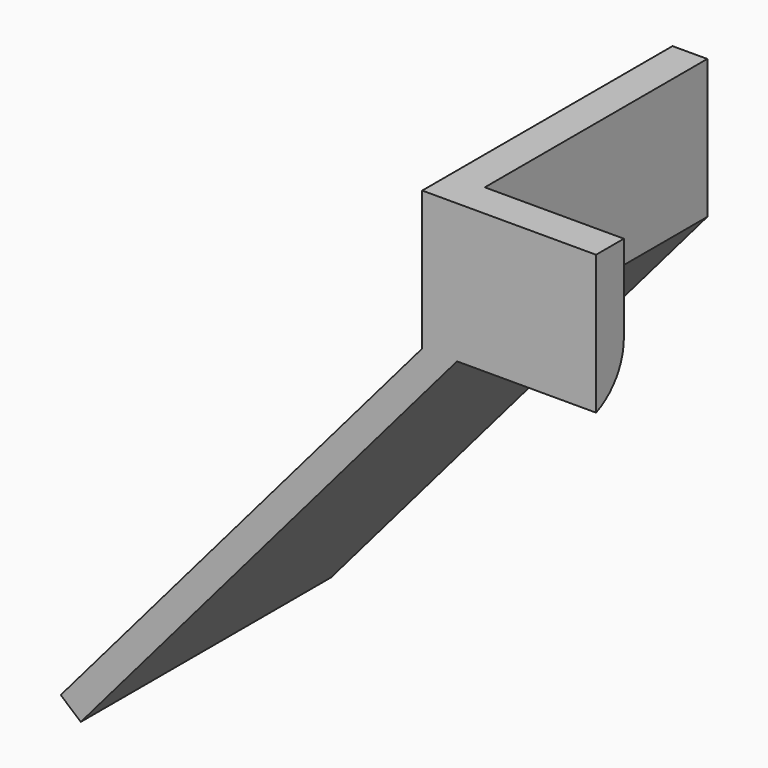
from build123d import *

# Parameters (mm, degrees)
F1_DEPTH    = 57.15
F2_W        = 6.35
F2_H        = 25.4
F3_DEPTH    = 25.4
F4_T1_DEPTH = 48.9464301965


# Not quite as in the source:
# - a fillet or chamfer that OpenCascade refuses, or shapes differently, is made with other operations: its cross-section is extruded or revolved along the edge and cut away or added


with BuildPart() as f1:
    # F0 (on Front) → F1 (new body)
    with BuildSketch(Plane.XZ):
        Polygon((36.6440817745, 56.0591582008), (30.2940817745, 56.0591582008), (30.2940817745, 30.6591582008), (-35.7496880067, -46.5469327059), (-32.0828693102, -49.6836091906), (36.6440817745, 30.6591582008), align=None)
    extrude(amount=F1_DEPTH)

    # F2 (on face) → F3 (join)
    with BuildSketch(Plane.YZ.offset(36.6440817745)):
        with Locations((-53.975, 43.3591582008)):
            Rectangle(F2_W, F2_H)
    extrude(amount=F3_DEPTH)

    # F4: fillet of radius 10.16 on 1 edges, made by hand

    # F4_s2 → F4_t1 (cut)
    with BuildSketch(Plane.YZ.offset(36.6440817745)):
        with BuildLine():
            ThreePointArc((-57.15, 30.6591582008), (-52.5357730325, 34.3981176165), (-50.8, 40.0777302794))
            Line((-50.8, 40.0777302794), (-50.8, 30.6591582008))
            Line((-50.8, 30.6591582008), (-57.15, 30.6591582008))
        make_face()
    extrude(amount=F4_T1_DEPTH, mode=Mode.SUBTRACT)


solid = f1.part
